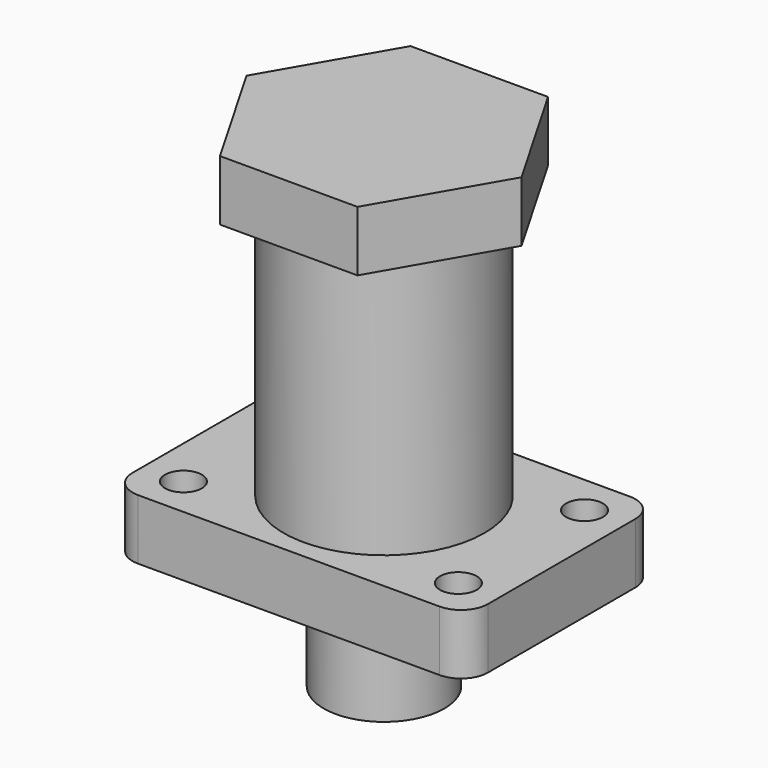
from build123d import *

# Parameters (mm, degrees)
F1_DEPTH  = 57.15
F2_R      = 95.25
F3_DEPTH  = 250.825
F5_DEPTH  = 57.15
F7_D      = 34.925
F8_R      = 57.15
F9_DEPTH  = 101.6
F11_D     = 57.15
F11_DEPTH = 406.4
F11_TIP   = 17.1695921887


with BuildPart() as f1:
    # F0 (on Top) → F1 (new body)
    with BuildSketch(Plane.XY):
        with BuildLine():
            Line((142.875, 112.7125), (-142.875, 112.7125))
            ThreePointArc((-142.875, 112.7125), (-160.8355122421, 105.2730122421), (-168.275, 87.3125))
            Line((-168.275, 87.3125), (-168.275, -87.3125))
            ThreePointArc((-168.275, -87.3125), (-160.8355122421, -105.2730122421), (-142.875, -112.7125))
            Line((-142.875, -112.7125), (142.875, -112.7125))
            ThreePointArc((142.875, -112.7125), (160.8355122421, -105.2730122421), (168.275, -87.3125))
            Line((168.275, -87.3125), (168.275, 87.3125))
            ThreePointArc((168.275, 87.3125), (160.8355122421, 105.2730122421), (142.875, 112.7125))
        make_face()
    extrude(amount=F1_DEPTH)

    # F2 (on face) → F3 (join)
    with BuildSketch(Plane.XY.offset(57.15)):
        Circle(F2_R)
    extrude(amount=F3_DEPTH)

    # F4 (on face) → F5 (join)
    with BuildSketch(Plane.XY.offset(307.975)):
        Polygon((65.11400916, 112.7807721496), (-65.11400916, 112.7807721496), (-130.2280183199, 0), (-65.11400916, -112.7807721496), (65.11400916, -112.7807721496), (130.2280183199, 0), align=None)
    extrude(amount=F5_DEPTH)

    # F7 (through all)
    with Locations(Plane(origin=(0, 0, 0), x_dir=(1, 0, 0), z_dir=(0, 0, -1))):
        with Locations((-130.175, 74.676), (-130.175, -74.676), (130.175, -74.676), (130.175, 74.676)):
            Hole(F7_D / 2)

    # F8 (on face) → F9 (join)
    with BuildSketch(Plane(origin=(0, 0, 0), x_dir=(1, 0, 0), z_dir=(0, 0, -1))):
        Circle(F8_R)
    extrude(amount=F9_DEPTH)

    # F11
    with Locations(Plane(origin=(0, 0, -101.6), x_dir=(1, 0, 0), z_dir=(0, 0, -1))):
        with Locations((0, 0)):
            Hole(F11_D / 2, depth=F11_DEPTH)
            with Locations((0, 0, -(F11_DEPTH + F11_TIP / 2))):  # 118° drill point
                Cone(0, F11_D / 2, F11_TIP, mode=Mode.SUBTRACT)


solid = f1.part
